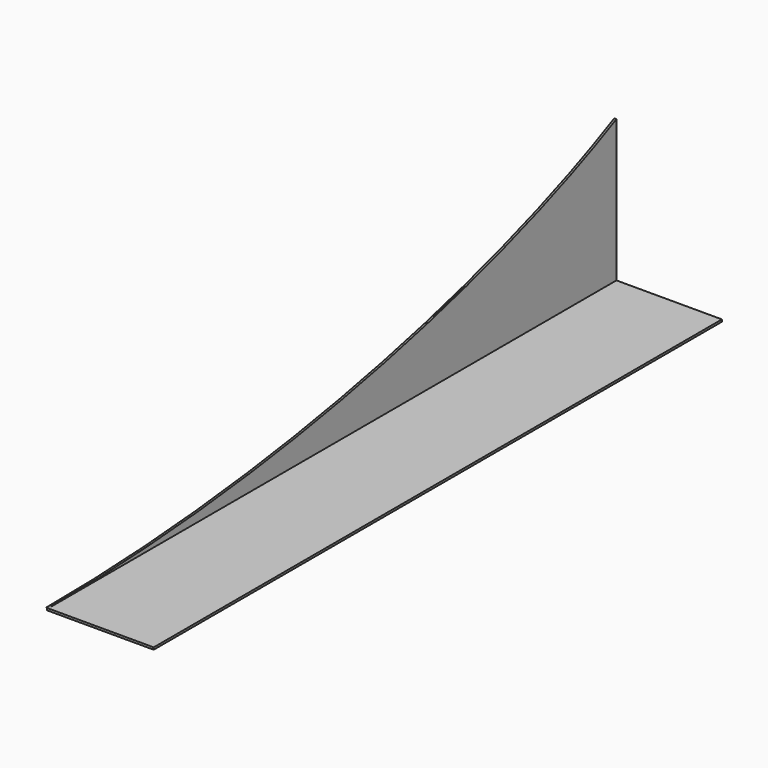
from build123d import *

# Parameters (mm, degrees)
F1_DEPTH = 1.5
F2_E1_W  = 1000
F2_E1_H  = 150
F3_DEPTH = 3


with BuildPart() as f1:
    # F0 (on Right) → F1 (new body, symmetric)
    with BuildSketch(Plane.YZ):
        with BuildLine():
            add(Edge.make_bspline(
                [(-507.5750658325, -64.4556317002), (-152.691480371, -64.4556317002), (239.9747440193, 9.7828772396), (492.4249341675, 135.5443682998)],
                knots=[0, 0, 0, 0, 1019.8039027186, 1019.8039027186, 1019.8039027186, 1019.8039027186], degree=3))
            Line((-507.5750658325, -64.4556317002), (492.4249341675, -64.4556317002))
            Line((492.4249341675, -64.4556317002), (492.4249341675, 135.5443682998))
        make_face()
    extrude(amount=F1_DEPTH, both=True)

    # F2_E1 (on explicit) → F3 (join)
    with BuildSketch(Plane(origin=(0, -507.5750658325, -64.4556317002), x_dir=(0, 1, 0), z_dir=(0, 0, -1))):
        with Locations((500, 75)):
            Rectangle(F2_E1_W, F2_E1_H)
    extrude(amount=F3_DEPTH)


solid = f1.part
